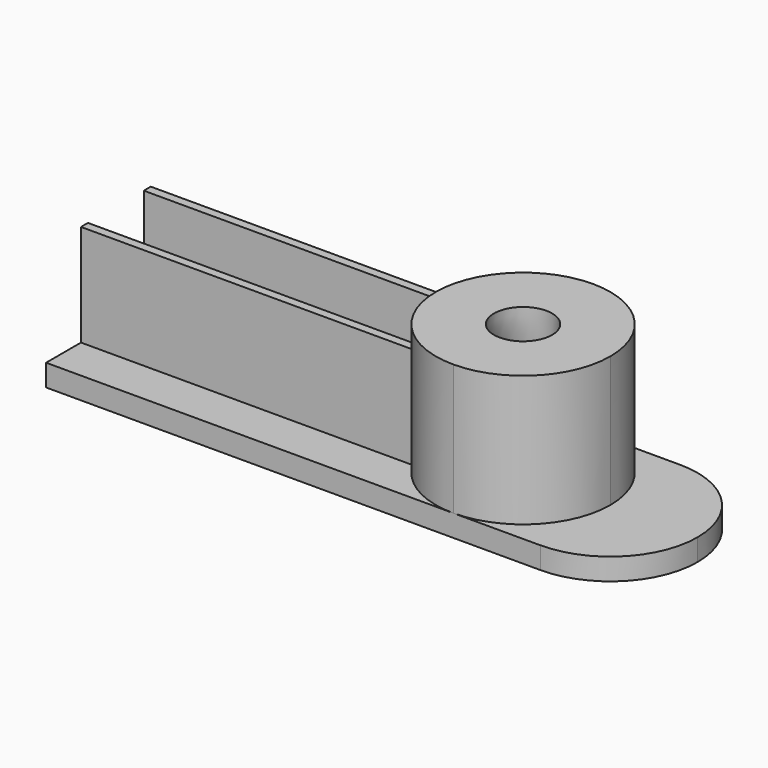
from build123d import *

# Parameters (mm, degrees)
F0_W     = 20
F0_H     = 6
F1_DEPTH = 0.75
F3_DEPTH = 4.5
F4_R     = 1
F6_R     = 2.99999
F8_DEPTH = 3.5


# Not quite as in the source:
# - a fillet or chamfer is up to 0.001 mm smaller than in the source, because OpenCascade refuses the exact size


with BuildPart() as f1:
    # F0 (on Top) → F1 (new body)
    with BuildSketch(Plane.XY):
        with Locations((-4, 0)):
            Rectangle(F0_W, F0_H)
    extrude(amount=F1_DEPTH)

    # F2 (on face) → F3 (join)
    with BuildSketch(Plane.XY.offset(0.75)):
        with BuildLine():
            ThreePointArc((0, -3), (2.1213203436, -2.1213203436), (3, 0))
            ThreePointArc((3, 0), (2.1213203436, 2.1213203436), (0, 3))
            ThreePointArc((0, 3), (-3, 0), (0, -3))
        make_face()
    extrude(amount=F3_DEPTH)

    # F4 (on face) → F5 (revolve, cut)
    with BuildSketch(Plane.XY.offset(5.25)):
        Circle(F4_R)
    revolve(axis=Axis((-3, -2.9594153166, 5.25), (0, -1, 0)), mode=Mode.SUBTRACT)

    # F6 (radius 3 in the source; OpenCascade refuses exactly that, so slightly less here)
    f6_edges = [f1.edges().sort_by_distance(p)[0] for p in [
        (6, -3, 0.375),
        (6, 3, 0.375),
    ]]
    fillet(f6_edges, radius=F6_R)

    # F7 (on face) → F8 (join)
    with BuildSketch(Plane.XY.offset(0.75)):
        with BuildLine():
            Line((-2.5980762114, 1.5), (-14, 1.5))
            Line((-14, 1.5), (-14, 1.2))
            Line((-14, 1.2), (-2.749545417, 1.2))
            ThreePointArc((-2.749545417, 1.2), (-2.6780149869, 1.3521226757), (-2.5980762114, 1.5))
        make_face()
        with BuildLine():
            Line((-2.749545417, -1.2), (-14, -1.2))
            Line((-14, -1.2), (-14, -1.5))
            Line((-14, -1.5), (-2.5980762114, -1.5))
            ThreePointArc((-2.5980762114, -1.5), (-2.6780149869, -1.3521226757), (-2.749545417, -1.2))
        make_face()
    extrude(amount=F8_DEPTH)


solid = f1.part
